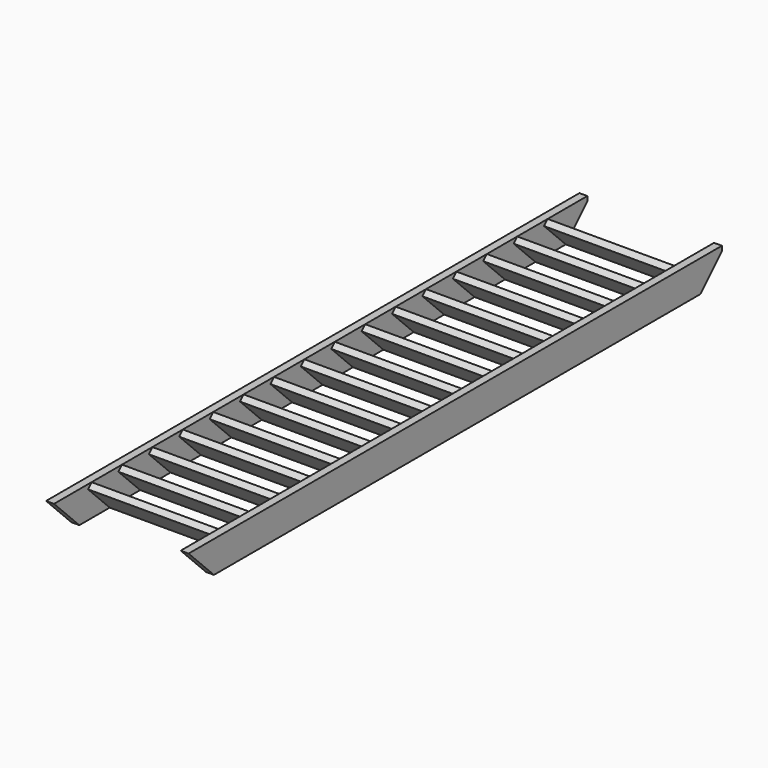
from build123d import *

# Parameters (mm, degrees)
F0_W     = 2.5
F0_H     = 210.5
F1_DEPTH = 10
F3_DEPTH = 41
F4_DEPTH = 3
F6_DEPTH = 4


with BuildPart() as f1:
    # F0 (on Top) → F1 (new body)
    with BuildSketch(Plane.XY):
        with Locations((-21.25, 0)):
            Rectangle(F0_W, F0_H)
    extrude(amount=F1_DEPTH)

    # F2 (on face) → F3 (join)
    with BuildSketch(Plane.YZ.offset(-20)):
        Polygon((-91.8357864376, 8.5857864376), (-83.25, 0), (-81.8357864376, 1.4142135624), (-90.4215728753, 10), align=None)
        Polygon((-79.8357864376, 8.5857864376), (-71.25, 0), (-69.8357864376, 1.4142135624), (-78.4215728753, 10), align=None)
        Polygon((-67.8357864376, 8.5857864376), (-59.25, 0), (-57.8357864376, 1.4142135624), (-66.4215728753, 10), align=None)
        Polygon((-55.8357864376, 8.5857864376), (-47.25, 0), (-45.8357864376, 1.4142135624), (-54.4215728753, 10), align=None)
        Polygon((-43.8357864376, 8.5857864376), (-35.25, 0), (-33.8357864376, 1.4142135624), (-42.4215728753, 10), align=None)
        Polygon((-31.8357864376, 8.5857864376), (-23.25, 0), (-21.8357864376, 1.4142135624), (-30.4215728753, 10), align=None)
        Polygon((-19.8357864376, 8.5857864376), (-11.25, 0), (-9.8357864376, 1.4142135624), (-18.4215728753, 10), align=None)
        Polygon((-7.8357864376, 8.5857864376), (0.75, 0), (2.1642135624, 1.4142135624), (-6.4215728753, 10), align=None)
        Polygon((4.1642135624, 8.5857864376), (12.75, 0), (14.1642135624, 1.4142135624), (5.5784271247, 10), align=None)
        Polygon((16.1642135624, 8.5857864376), (24.75, 0), (26.1642135624, 1.4142135624), (17.5784271247, 10), align=None)
        Polygon((28.1642135624, 8.5857864376), (36.75, 0), (38.1642135624, 1.4142135624), (29.5784271247, 10), align=None)
        Polygon((40.1642135624, 8.5857864376), (48.75, 0), (50.1642135624, 1.4142135624), (41.5784271247, 10), align=None)
        Polygon((52.1642135624, 8.5857864376), (60.75, 0), (62.1642135624, 1.4142135624), (53.5784271247, 10), align=None)
        Polygon((64.1642135624, 8.5857864376), (72.75, 0), (74.1642135624, 1.4142135624), (65.5784271247, 10), align=None)
        Polygon((76.1642135624, 8.5857864376), (84.75, 0), (86.1642135624, 1.4142135624), (77.5784271247, 10), align=None)
        Polygon((88.1642135624, 8.5857864376), (96.75, 0), (98.1642135624, 1.4142135624), (89.5784271247, 10), align=None)
    extrude(amount=F3_DEPTH)

    # F2 (on face) → F4 (cut)
    with BuildSketch(Plane.YZ.offset(-20)):
        Polygon((98.1642135624, 1.4142135624), (96.75, 0), (105.25, 0), (105.25, 8.5), align=None)
        Polygon((-105.25, 10), (-105.25, 0), (-95.25, 0), align=None)
    extrude(amount=-F4_DEPTH, mode=Mode.SUBTRACT)


with BuildPart() as f1b:
    # F0 (on Top) → F1, piece 2 (new body)
    with BuildSketch(Plane.XY):
        with Locations((21.25, 0)):
            Rectangle(F0_W, F0_H)
    extrude(amount=F1_DEPTH)

    # F5 (on face) → F6 (cut)
    with BuildSketch(Plane(origin=(20, 0, 0), x_dir=(0, -1, 0), z_dir=(-1, 0, 0))):
        Polygon((105.25, 10), (95.25, 0), (105.25, 0), align=None)
        Polygon((-96.75, 0), (-105.25, 8.5), (-105.25, 0), align=None)
    extrude(amount=-F6_DEPTH, mode=Mode.SUBTRACT)


solid = Compound([f1.part, f1b.part])
